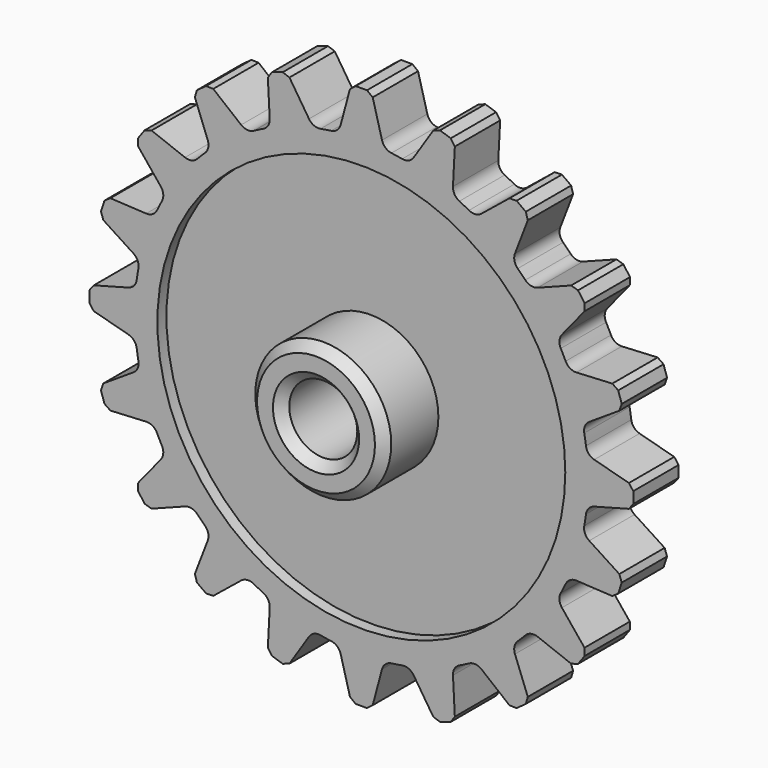
from build123d import *

# Parameters (mm, degrees)
F0_R            = 100
F1_DEPTH        = 25
F3_DEPTH        = 25
F3_COPIES_COUNT = 20
F4_R            = 5
F5_SIZE         = 2
F6_R            = 90
F7_DEPTH        = 5
F8_R            = 30
F9_DEPTH        = 30
F10_R           = 15
F11_DEPTH       = 50.001
F12_SIZE        = 4


# Not quite as in the source:
# - a pattern or mirror of a feature is missing from the dataset's text; its kind, count and spacing are read off the source's solid
# - a feature names something its author has since deleted; it is built from what else it names


with BuildPart() as f1:
    # F0 (on Front) → F1 (new body)
    with BuildSketch(Plane.XZ):
        Circle(F0_R)
    extrude(amount=F1_DEPTH)

    # F2 (on face) → F3 (join)
    with BuildSketch(Plane.XZ.offset(25)):
        Polygon((-4.5, 120), (-9.9931095726, 99.4994359837), (9.9931095726, 99.4994359837), (4.5, 120), align=None)
    f3 = extrude(amount=-F3_DEPTH)

    # F3_copies: F3 ×20 about axis
    f3_copies_axis = Axis((0, 0, 0), (0, 1, 0))
    for i in range(1, F3_COPIES_COUNT):
        add(f3.rotate(f3_copies_axis, i * 360 / F3_COPIES_COUNT))

    # F4
    f4_edges = [f1.edges().sort_by_distance(p)[0] for p in [
        (9.99311, -12.5, 99.499436),
        (-9.99311, -12.5, 99.499436),
        (-21.243005, -12.5, 97.717628),
        (97.717628, -12.5, 21.243005),
        (99.499436, -12.5, 9.99311),
        (99.499436, -12.5, -9.99311),
        (97.717628, -12.5, -21.243005),
        (91.541546, -12.5, -40.251029),
        (86.370537, -12.5, -50.399706),
        (74.622932, -12.5, -66.568897),
        (66.568897, -12.5, -74.622932),
        (50.399706, -12.5, -86.370537),
        (40.251029, -12.5, -91.541546),
        (21.243005, -12.5, -97.717628),
        (9.99311, -12.5, -99.499436),
        (-9.99311, -12.5, -99.499436),
        (-21.243005, -12.5, -97.717628),
        (-40.251029, -12.5, -91.541546),
        (-50.399706, -12.5, -86.370537),
        (-66.568897, -12.5, -74.622932),
        (-74.622932, -12.5, -66.568897),
        (-86.370537, -12.5, -50.399706),
        (-91.541546, -12.5, -40.251029),
        (-97.717628, -12.5, -21.243005),
        (-99.499436, -12.5, -9.99311),
        (-99.499436, -12.5, 9.99311),
        (-97.717628, -12.5, 21.243005),
        (-91.541546, -12.5, 40.251029),
        (-86.370537, -12.5, 50.399706),
        (-74.622932, -12.5, 66.568897),
        (-66.568897, -12.5, 74.622932),
        (-50.399706, -12.5, 86.370537),
        (-40.251029, -12.5, 91.541546),
        (21.243005, -12.5, 97.717628),
        (40.251029, -12.5, 91.541546),
        (50.399706, -12.5, 86.370537),
        (66.568897, -12.5, 74.622932),
        (74.622932, -12.5, 66.568897),
        (86.370537, -12.5, 50.399706),
        (91.541546, -12.5, 40.251029),
    ]]
    fillet(f4_edges, radius=F4_R)

    # F5
    f5_edges = [f1.edges().sort_by_distance(p)[0] for p in [
        (4.5, -12.5, 120),
        (-4.5, -12.5, 120),
        (115.517358, -12.5, 32.802285),
        (112.736205, -12.5, 41.361794),
        (120, -12.5, 4.5),
        (120, -12.5, -4.5),
        (99.727073, -12.5, 66.893654),
        (94.437006, -12.5, 74.174807),
        (115.517358, -12.5, -32.802285),
        (112.736205, -12.5, -41.361794),
        (74.174807, -12.5, 94.437006),
        (66.893654, -12.5, 99.727073),
        (99.727073, -12.5, -66.893654),
        (94.437006, -12.5, -74.174807),
        (41.361794, -12.5, 112.736205),
        (32.802285, -12.5, 115.517358),
        (74.174807, -12.5, -94.437006),
        (66.893654, -12.5, -99.727073),
        (41.361794, -12.5, -112.736205),
        (32.802285, -12.5, -115.517358),
        (-32.802285, -12.5, 115.517358),
        (-41.361794, -12.5, 112.736205),
        (4.5, -12.5, -120),
        (-4.5, -12.5, -120),
        (-66.893654, -12.5, 99.727073),
        (-74.174807, -12.5, 94.437006),
        (-32.802285, -12.5, -115.517358),
        (-41.361794, -12.5, -112.736205),
        (-94.437006, -12.5, 74.174807),
        (-99.727073, -12.5, 66.893654),
        (-66.893654, -12.5, -99.727073),
        (-74.174807, -12.5, -94.437006),
        (-112.736205, -12.5, 41.361794),
        (-115.517358, -12.5, 32.802285),
        (-94.437006, -12.5, -74.174807),
        (-99.727073, -12.5, -66.893654),
        (-120, -12.5, 4.5),
        (-120, -12.5, -4.5),
        (-112.736205, -12.5, -41.361794),
        (-115.517358, -12.5, -32.802285),
    ]]
    chamfer(f5_edges, length=F5_SIZE)

    # F6 (on face) → F7 (cut)
    with BuildSketch(Plane.XZ.offset(25)):
        Circle(F6_R)
    extrude(amount=-F7_DEPTH, mode=Mode.SUBTRACT)

    # F8 (on face) → F9 (join)
    with BuildSketch(Plane.XZ.offset(20)):
        Circle(F8_R)
    extrude(amount=F9_DEPTH)

    # F10 (on face) → F11 (cut, through all)
    with BuildSketch(Plane.XZ.offset(50)):
        Circle(F10_R)
    extrude(amount=-F11_DEPTH, mode=Mode.SUBTRACT)

    # F12
    f12_edges = [f1.edges().sort_by_distance(p)[0] for p in [
        (-15, -50, 0),
        (-30, -50, 0),
    ]]
    chamfer(f12_edges, length=F12_SIZE)


solid = f1.part
